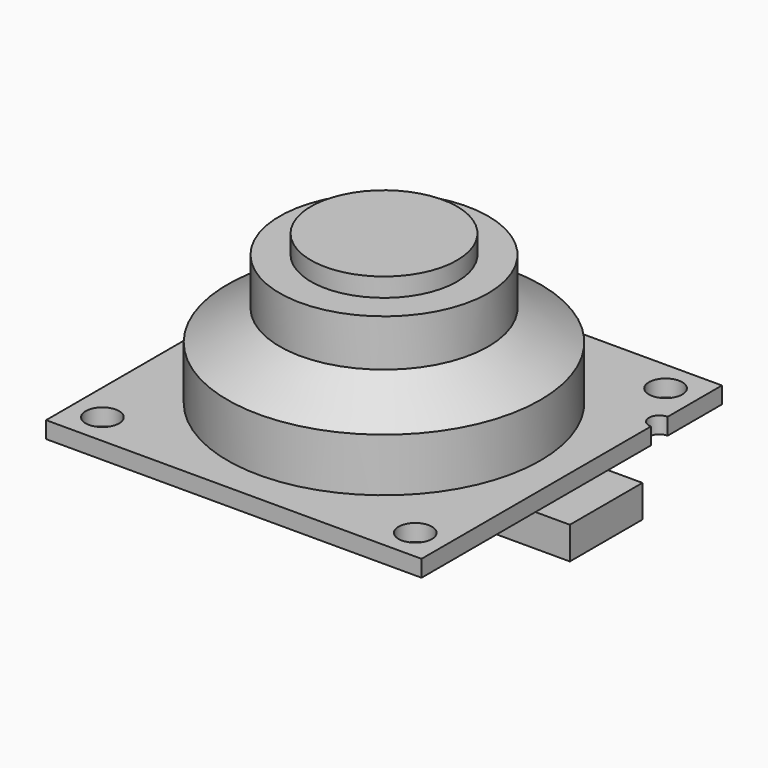
from build123d import *

# Parameters (mm, degrees)
F0_R     = 1.6
F0_W     = 2
F0_H     = 2
F0_W_2   = 13.7
F0_H_2   = 2.9
F0_W_3   = 7.4758231461
F0_H_3   = 8.7
F1_DEPTH = 1.6
F2_DEPTH = 4
F0_W_4   = 3.3
F3_DEPTH = 3.1
F4_DEPTH = 2
F5_R     = 15
F5_R_2   = 10
F6_DEPTH = 8
F7_DEPTH = 12.5
F8_SIZE2 = 2.886741
F8_SIZE  = 4.99999
F5_R_3   = 7
F9_DEPTH = 14.3


# Not quite as in the source:
# - a fillet or chamfer is up to 0.001 mm smaller than in the source, because OpenCascade refuses the exact size


with BuildPart() as f1:
    # F0 (on Top) → F1 (new body)
    with BuildSketch(Plane.XY):
        with BuildLine():
            Line((-18, -18), (18, -18))
            Line((18, -18), (18, -4.35))
            Line((18, -4.35), (10.5241768539, -4.35))
            Line((10.5241768539, -4.35), (10.5241768539, 4.35))
            Line((10.5241768539, 4.35), (18, 4.35))
            Line((18, 4.35), (18, 9.5))
            ThreePointArc((18, 9.5), (17, 10.5), (18, 11.5))
            Line((18, 11.5), (18, 18))
            Line((18, 18), (-18, 18))
            Line((-18, 18), (-18, -18))
        make_face()
        with Locations((-15, -15)):
            Circle(F0_R, mode=Mode.SUBTRACT)
        with Locations((-15.5, -10.5)):
            Rectangle(F0_W, F0_H, mode=Mode.SUBTRACT)
        with Locations((15, -15)):
            Circle(F0_R, mode=Mode.SUBTRACT)
        with Locations((-15, 15)):
            Circle(F0_R, mode=Mode.SUBTRACT)
        with Locations((0, 15.9)):
            Rectangle(F0_W_2, F0_H_2, mode=Mode.SUBTRACT)
        with Locations((15, 15)):
            Circle(F0_R, mode=Mode.SUBTRACT)
        with Locations((0, 15.9)):
            Rectangle(F0_W_2, F0_H_2)
        with Locations((-15.5, -10.5)):
            Rectangle(F0_W, F0_H)
        with Locations((14.2620884269, 0)):
            Rectangle(F0_W_3, F0_H_3)
    extrude(amount=F1_DEPTH)

    # F0 (on Top) → F2 (join)
    with BuildSketch(Plane.XY):
        with Locations((0, 15.9)):
            Rectangle(F0_W_2, F0_H_2)
    extrude(amount=-F2_DEPTH)

    # F0 (on Top) → F3 (join)
    with BuildSketch(Plane.XY):
        with Locations((19.65, 0)):
            Rectangle(F0_W_4, F0_H_3)
        with Locations((14.2620884269, 0)):
            Rectangle(F0_W_3, F0_H_3)
    extrude(amount=-F3_DEPTH)

    # F0 (on Top) → F4 (join)
    with BuildSketch(Plane.XY):
        with Locations((-15.5, -10.5)):
            Rectangle(F0_W, F0_H)
    extrude(amount=-F4_DEPTH)

    # F5 (on face) → F6 (join)
    with BuildSketch(Plane.XY.offset(1.6)):
        Circle(F5_R)
        Circle(F5_R_2, mode=Mode.SUBTRACT)
    extrude(amount=F6_DEPTH)

    # F7 (add): a face of the model
    f7_faces = [f1.faces().sort_by_distance(p)[0] for p in [
        (0, 0, 1.6),
    ]]
    extrude(f7_faces, amount=F7_DEPTH)

    # F8 (size 5 and 2.8867513459 in the source; OpenCascade refuses exactly that, so slightly less here)
    f8_edges = [f1.edges().sort_by_distance(p)[0] for p in [
        (-15, 0, 9.6),
    ]]
    f8_side = f1.faces().sort_by_distance((-14.575736, 0, 9.6))[0]
    chamfer(f8_edges, length=F8_SIZE, length2=F8_SIZE2, reference=f8_side)

    # F5 (on face) → F9 (join)
    with BuildSketch(Plane.XY.offset(1.6)):
        Circle(F5_R_3)
    extrude(amount=F9_DEPTH)


solid = f1.part
